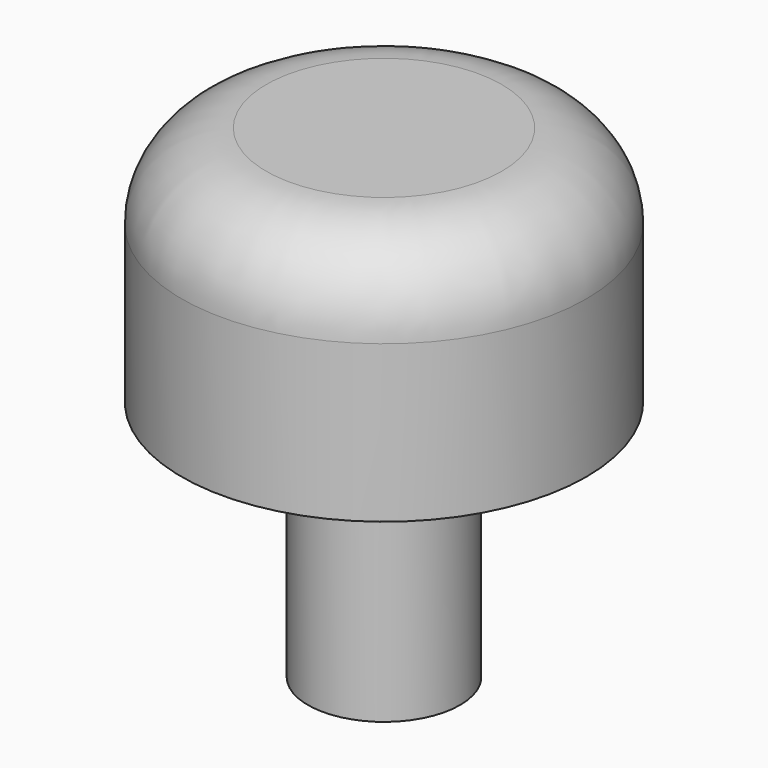
from build123d import *

# Parameters (mm, degrees)
F0_R     = 23.9
F1_DEPTH = 28.5
F2_R     = 8.98
F3_DEPTH = 28.575
F4_R     = 10


# Not quite as in the source:
# - a length typed as a fraction of an inch, garbled in the dataset ("3 / 203.2 mm" for 3/8 in), is restored


with BuildPart() as f1:
    # F0 (on Top) → F1 (new body)
    with BuildSketch(Plane.XY):
        Circle(F0_R)
    extrude(amount=F1_DEPTH)

    # F2 (on face) → F3 (join)
    with BuildSketch(Plane(origin=(0, 0, 0), x_dir=(1, 0, 0), z_dir=(0, 0, -1))):
        Circle(F2_R)
    extrude(amount=F3_DEPTH)

    # F4
    f4_edges = [f1.edges().sort_by_distance(p)[0] for p in [
        (-23.9, 0, 28.5),
    ]]
    fillet(f4_edges, radius=F4_R)


solid = f1.part
